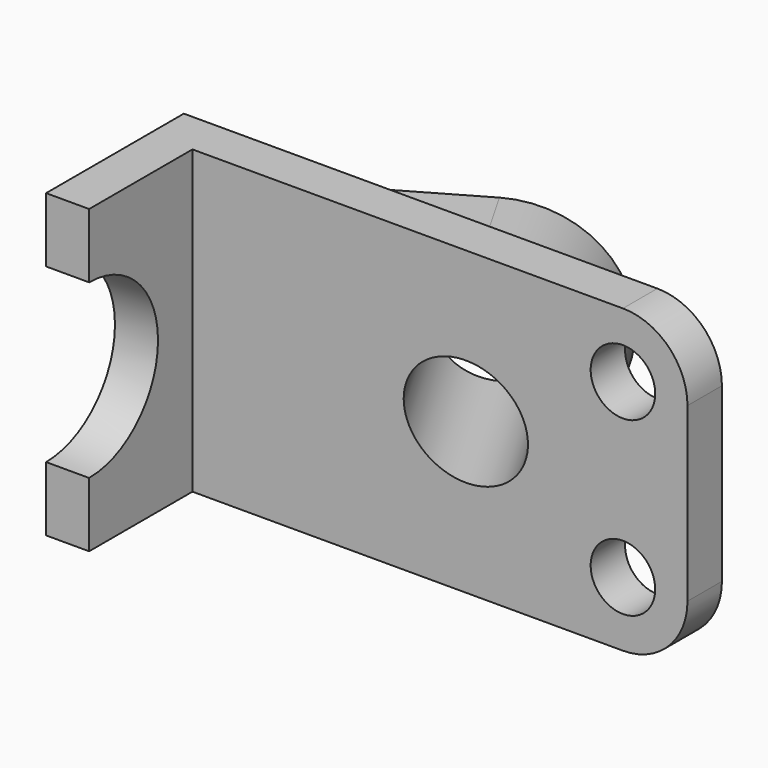
from build123d import *

# Parameters (mm, degrees)
F1_DEPTH  = 70
F4_DEPTH  = 50
F6_REACH  = 161.8626818177
F7_R      = 12.5
F8_DEPTH  = 92.1420161514
F9_R      = 15
F10_R     = 7.5
F11_DEPTH = 25
F12_R     = 20
F13_DEPTH = 25


with BuildPart() as f1:
    # F0 (on Top) → F1 (new body)
    with BuildSketch(Plane.XY):
        Polygon((0, -10), (0, 0), (-125, 0), (-125, -40), (-115, -40), (-115, -10), align=None)
    extrude(amount=F1_DEPTH)

    # F3 (on offset) → F4 (join)
    with BuildSketch(Plane.XY.offset(60)):
        Polygon((-115, 0), (-28.3974596216, 0), (-50.0480947162, 37.5), align=None)
    extrude(amount=-F4_DEPTH)

    f6_end = Plane(origin=(-53.4880513164, 0, 35), x_dir=(0, 0, 1), z_dir=(0, 1, 0))
    # F5 (on face) → F6 (cut, up to a plane its end follows)
    with BuildSketch(Plane(origin=(-28.75, 49.7964607176, 0), x_dir=(-0.8660254038, -0.5, 0), z_dir=(-0.5, 0.8660254038, 0))):
        with BuildLine():
            ThreePointArc((49.5929214352, 10), (24.5929214352, 35), (49.5929214352, 60))
            Line((49.5929214352, 60), (49.5929214352, 65.1633962989))
            Line((49.5929214352, 65.1633962989), (18.7135729939, 65.1633962989))
            Line((18.7135729939, 65.1633962989), (18.7135729939, 2.6539005339))
            Line((18.7135729939, 2.6539005339), (49.5929214352, 2.6539005339))
            Line((49.5929214352, 2.6539005339), (49.5929214352, 10))
        make_face()
    f6_long = extrude(amount=-F6_REACH, mode=Mode.PRIVATE)
    add(split(f6_long, bisect_by=f6_end, keep=Keep.TOP, mode=Mode.PRIVATE), mode=Mode.SUBTRACT)

    # F7 (on face) → F8 (cut, through all)
    with BuildSketch(Plane(origin=(-28.75, 49.7964607176, 0), x_dir=(-0.8660254038, -0.5, 0), z_dir=(-0.5, 0.8660254038, 0))):
        with Locations((49.5929214352, 35)):
            Circle(F7_R)
    extrude(amount=-F8_DEPTH, mode=Mode.SUBTRACT)

    # F9
    f9_edges = [f1.edges().sort_by_distance(p)[0] for p in [
        (0, -5, 70),
        (0, -5, 0),
    ]]
    fillet(f9_edges, radius=F9_R)

    # F10 (on face) → F11 (cut)
    with BuildSketch(Plane(origin=(0, 0, 0), x_dir=(-1, 0, 0), z_dir=(0, 1, 0))):
        with Locations((15, 15)):
            Circle(F10_R)
        with Locations((15, 55)):
            Circle(F10_R)
    extrude(amount=-F11_DEPTH, mode=Mode.SUBTRACT)

    # F12 (on face) → F13 (cut)
    with BuildSketch(Plane(origin=(-125, 0, 0), x_dir=(0, -1, 0), z_dir=(-1, 0, 0))):
        with Locations((40, 35)):
            Circle(F12_R)
    extrude(amount=-F13_DEPTH, mode=Mode.SUBTRACT)


solid = f1.part
